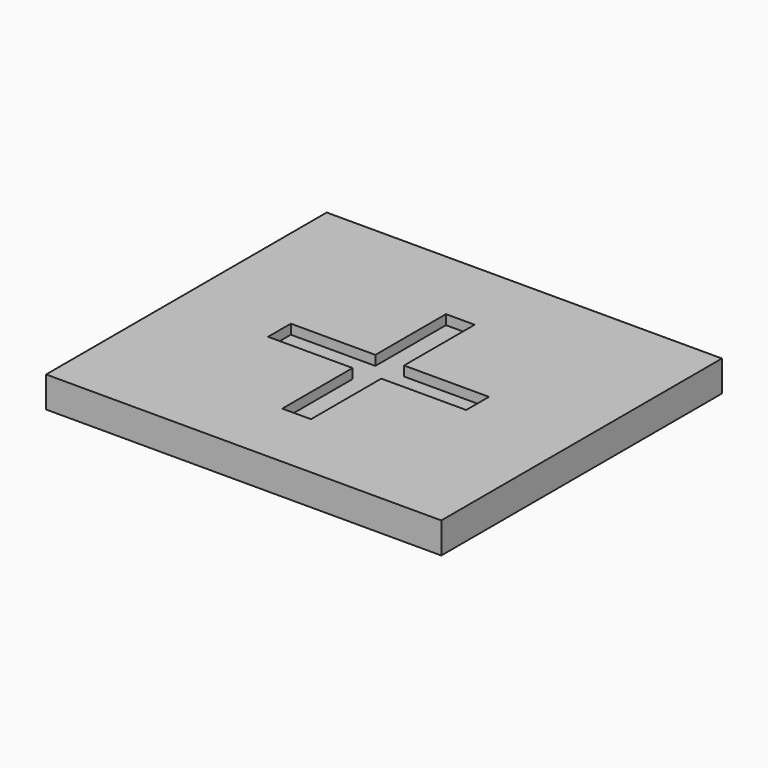
from build123d import *

# Parameters (mm, degrees)
F0_W         = 40.64
F0_H         = 36.068
F1_DEPTH     = 3.175
F2_TEXT_SIZE = 43.4304034197
F3_DEPTH     = 1


# Not quite as in the source:
# - Text() gives the source's letters only with a copy of the font that has no kerning and outlines rounded to 1/6400 em; it was checked with that copy


with BuildPart() as f1:
    # F0 (on Top) → F1 (new body)
    with BuildSketch(Plane.XY):
        Rectangle(F0_W, F0_H)
    extrude(amount=F1_DEPTH)

    # F2 (on face) → F3 (cut)
    with BuildSketch(Plane.XY.offset(3.175)):
        with Locations((-12.7, -15.6349452311)):
            Text('+', F2_TEXT_SIZE, font='Open Sans', text_align=(TextAlign.LEFT, TextAlign.BOTTOM))
    extrude(amount=-F3_DEPTH, mode=Mode.SUBTRACT)


solid = f1.part
